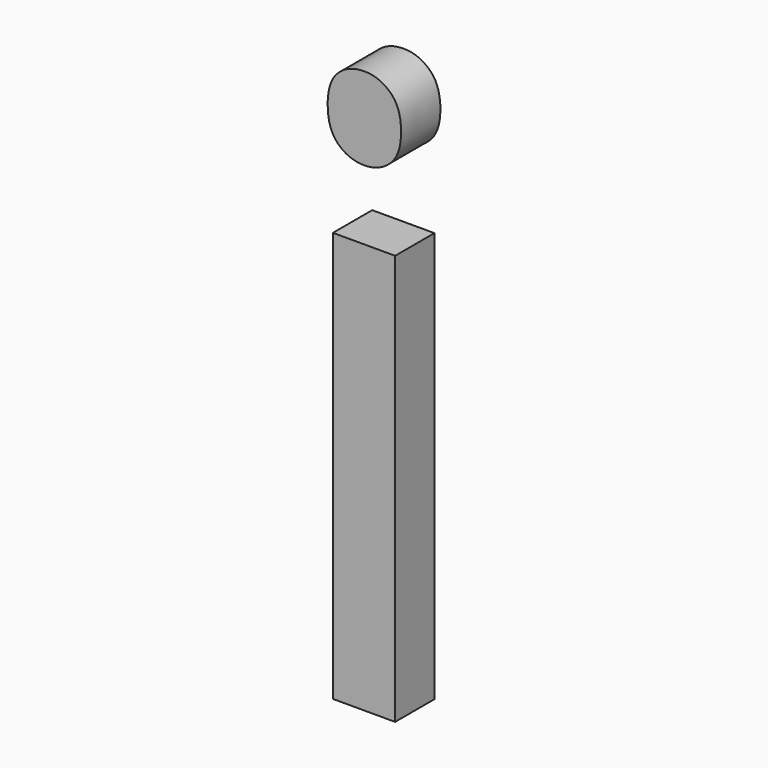
from build123d import *

# Parameters (mm, degrees)
F0_TEXT_SIZE = 39.6572053432
F1_DEPTH     = 2.54


# Not quite as in the source:
# - Text() gives the source's letters only with a copy of the font that has no kerning and outlines rounded to 1/6400 em; it was checked with that copy


with BuildPart() as f1:
    # F0 (on Front) → F1 (new body)
    with BuildSketch(Plane.XZ):
        with Locations((-9.5053364057, 0)):
            Text('i', F0_TEXT_SIZE, font='Open Sans', text_align=(TextAlign.LEFT, TextAlign.BOTTOM))
    extrude(amount=F1_DEPTH)


solid = f1.part
